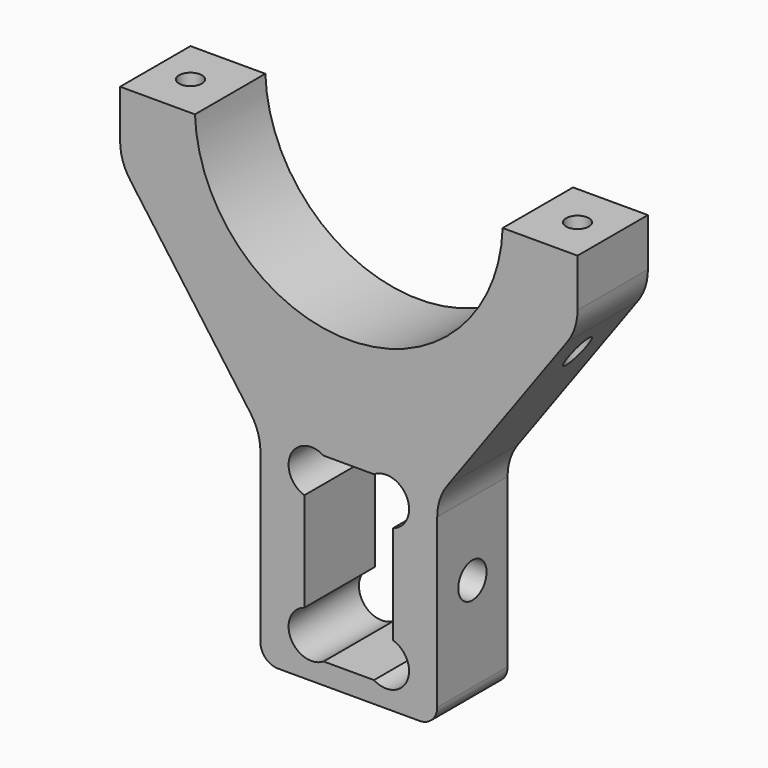
from build123d import *

# Parameters (mm, degrees)
F0_W     = 12.827
F0_H     = 26.162
F1_DEPTH = 6.35
F3_D     = 5.1054
F3_DEPTH = 26.6075
F5_D     = 3.3
F6_R     = 3.302
F7_DEPTH = 12.701
F8_R     = 2.54
F9_R     = 7.62
F10_R    = 7.62


# Not quite as in the source:
# - a pattern or mirror of a feature is missing from the dataset's text; its kind, count and spacing are read off the source's solid


with BuildPart() as f1:
    # F0 (on Front) → F1 (new body, symmetric)
    with BuildSketch(Plane.XZ):
        with BuildLine():
            Line((-12.7635, -29.21), (12.7635, -29.21))
            Line((12.7635, -29.21), (12.7635, 0))
            Line((12.7635, 0), (33.02, 27.94))
            Line((33.02, 27.94), (33.02, 37.338))
            Line((33.02, 37.338), (22.2119333017, 37.338))
            ThreePointArc((22.2119333017, 37.338), (0, 15.875), (-22.2119333017, 37.338))
            Line((-22.2119333017, 37.338), (-33.02, 37.338))
            Line((-33.02, 37.338), (-33.02, 27.94))
            Line((-33.02, 27.94), (-12.7635, 0))
            Line((-12.7635, 0), (-12.7635, -29.21))
        make_face()
        with Locations((0, -13.081)):
            Rectangle(F0_W, F0_H, mode=Mode.SUBTRACT)
    extrude(amount=F1_DEPTH, both=True)

    # F3 (through all, one way)
    with BuildSketch(Plane(origin=(6.4135, 0, 0), x_dir=(0, -1, 0), z_dir=(-1, 0, 0))):
        with Locations((0, -13.081)):
            Circle(F3_D / 2)
    extrude(amount=-F3_DEPTH, mode=Mode.SUBTRACT)

    # F5 (through all)
    with Locations(Plane.XY.offset(37.338)):
        with Locations((-27.94, 0)):
            f5 = Hole(F5_D / 2)

    # F5_copies: F5 across plane
    add(f5.mirror(Plane(origin=(6e-06, 0, 0), x_dir=(0, 0, 1), z_dir=(1, 0, 0))), mode=Mode.SUBTRACT)

    # F6 (on face) → F7 (cut, through all)
    with BuildSketch(Plane.XZ.offset(6.35)):
        with Locations((-5.3975, -2.794)):
            Circle(F6_R)
        with Locations((-5.3975, -23.368)):
            Circle(F6_R)
        with Locations((5.3975, -2.794)):
            Circle(F6_R)
        with Locations((5.3975, -23.368)):
            Circle(F6_R)
    extrude(amount=-F7_DEPTH, mode=Mode.SUBTRACT)

    # F8
    f8_edges = [f1.edges().sort_by_distance(p)[0] for p in [
        (12.7635, 0, -29.21),
        (-12.7635, 0, -29.21),
    ]]
    fillet(f8_edges, radius=F8_R)

    # F9
    f9_edges = [f1.edges().sort_by_distance(p)[0] for p in [
        (12.7635, 0, 0),
        (-12.7635, 0, 0),
    ]]
    fillet(f9_edges, radius=F9_R)

    # F10
    f10_edges = [f1.edges().sort_by_distance(p)[0] for p in [
        (33.02, 0, 27.94),
        (-33.02, 0, 27.94),
    ]]
    fillet(f10_edges, radius=F10_R)


solid = f1.part
